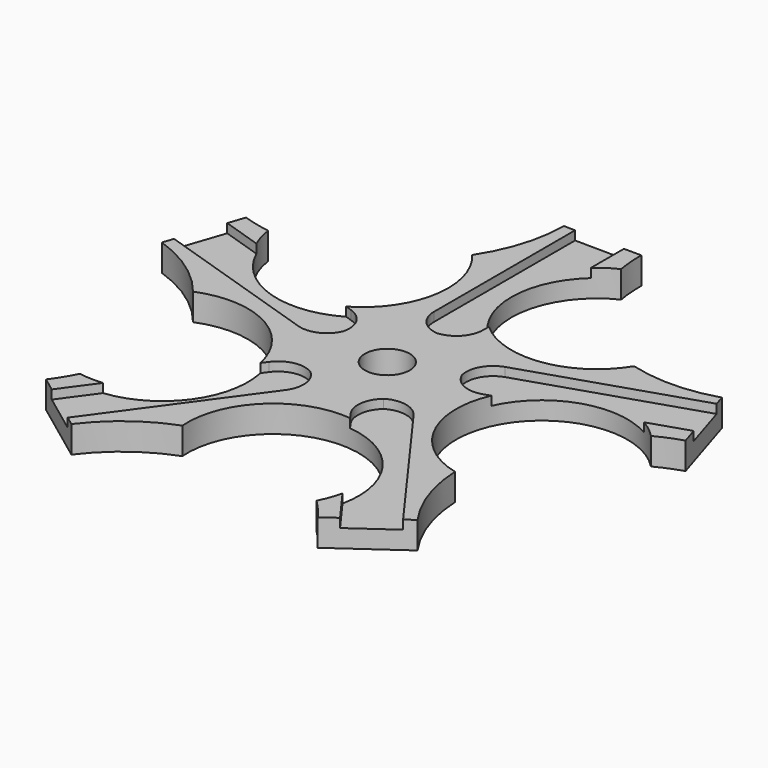
from build123d import *

# Parameters (mm, degrees)
F0_R        = 2.5
F1_DEPTH    = 3
F3_DEPTH    = 1
F4_T1_DEPTH = 1


# Not quite as in the source:
# - a fillet or chamfer that OpenCascade refuses, or shapes differently, is made with other operations: its cross-section is extruded or revolved along the edge and cut away or added


with BuildPart() as f1:
    # F0 (on Top) → F1 (new body)
    with BuildSketch(Plane.XY):
        with BuildLine():
            Line((42.1995138221, 67.0275468757), (33.4926469464, 67.1294207869))
            ThreePointArc((33.4926469464, 67.1294207869), (32.7404851321, 62.3046461892), (30.658157874, 57.8878475177))
            ThreePointArc((30.658157874, 57.8878475177), (27.294204133, 42.9798709067), (13.9152540739, 50.3668626301))
            ThreePointArc((13.9152540739, 50.3668626301), (12.375918121, 50.6607466073), (10.86986377, 51.0940170307))
            Line((10.86986377, 51.0940170307), (8.0824060906, 42.844775322))
            ThreePointArc((8.0824060906, 42.844775322), (12.4386086282, 40.6384895823), (15.9957592753, 37.2932128243))
            ThreePointArc((15.9957592753, 37.2932128243), (29.1345687017, 29.4870845738), (17.9747991522, 19.0456529188))
            ThreePointArc((17.9747991522, 19.0456529188), (17.2196179112, 17.6724725733), (16.3421568627, 16.3740176929))
            Line((16.3421568627, 16.3740176929), (23.3262801503, 11.1738320243))
            ThreePointArc((23.3262801503, 11.1738320243), (26.7707231948, 14.6350470461), (31.0514904559, 16.9843509793))
            ThreePointArc((31.0514904559, 16.9843509793), (42.5356749941, 27.0678750109), (49.017508165, 13.2277236335))
            ThreePointArc((49.017508165, 13.2277236335), (50.0901164433, 12.0851675302), (51.0538700425, 10.8494078578))
            Line((51.0538700425, 10.8494078578), (58.1577532953, 15.8847580755))
            ThreePointArc((58.1577532953, 15.8847580755), (55.9303336315, 20.230192341), (55.0188426496, 25.0274187796))
            ThreePointArc((55.0188426496, 25.0274187796), (48.977649601, 39.065507608), (64.1434123595, 40.9532553024))
            ThreePointArc((64.1434123595, 40.9532553024), (65.5615019731, 41.620297142), (67.0345955027, 42.1550105429))
            Line((67.0345955027, 42.1550105429), (64.4409135174, 50.4672137913))
            ThreePointArc((64.4409135174, 50.4672137913), (59.6198494134, 49.6916248415), (54.7757497452, 50.307169899))
            ThreePointArc((54.7757497452, 50.307169899), (39.5579025703, 48.8996619005), (42.4490262494, 63.9065055152))
            ThreePointArc((42.4490262494, 63.9065055152), (42.2528455514, 65.4613161473), (42.1995138221, 67.0275468757))
        make_face()
        with Locations((37.5, 37.5)):
            Circle(F0_R, mode=Mode.SUBTRACT)
    extrude(amount=F1_DEPTH)

    # F2 (on face) → F3 (cut)
    with BuildSketch(Plane.XY.offset(3)):
        Polygon((40.25, 67.1147092408), (34.75, 67.1147092408), (40.25, 67.0503569865), align=None)
        with BuildLine():
            Line((31.7569283434, 42.2575582148), (28.1635644564, 43.4251129174))
            ThreePointArc((28.1635644564, 43.4251129174), (20.4254111601, 42.6084822131), (14.6451171229, 47.8175227185))
            Line((14.6451171229, 47.8175227185), (10.2457371637, 49.2469679185))
            Line((10.2457371637, 49.2469679185), (8.4849410638, 44.0360430191))
            Line((8.4849410638, 44.0360430191), (30.0573348743, 37.0267473751))
            Line((30.0573348743, 37.0267473751), (31.7569283434, 42.2575582148))
        make_face()
        with BuildLine():
            Line((31.2005865164, 33.5081806175), (28.9797655003, 30.4514827223))
            ThreePointArc((28.9797655003, 30.4514827223), (27.3652065793, 22.8397088401), (20.6249055731, 18.9520045705))
            Line((20.6249055731, 18.9520045705), (17.9059392288, 15.2096684519))
            Line((17.9059392288, 15.2096684519), (22.3177073919, 11.9247874969))
            Line((22.3177073919, 11.9247874969), (35.6501799855, 30.2753617299))
            Line((35.6501799855, 30.2753617299), (31.2005865164, 33.5081806175))
        make_face()
        with BuildLine():
            Line((52.6444673021, 11.9768495643), (57.1318860772, 15.1576063845))
            Line((57.1318860772, 15.1576063845), (43.7994134836, 33.5081806175))
            Line((43.7994134836, 33.5081806175), (39.3498200145, 30.2753617299))
            Line((39.3498200145, 30.2753617299), (41.5706410307, 27.2186638347))
            ThreePointArc((41.5706410307, 27.2186638347), (48.3109420369, 23.3309595651), (49.9255009579, 15.7191856828))
            Line((49.9255009579, 15.7191856828), (52.6444673021, 11.9768495643))
        make_face()
        with BuildLine():
            Line((66.4538563054, 44.0161570789), (64.8154654671, 49.2668538587))
            Line((64.8154654671, 49.2668538587), (43.2430716566, 42.2575582148))
            Line((43.2430716566, 42.2575582148), (44.9426651257, 37.0267473751))
            Line((44.9426651257, 37.0267473751), (48.5360290127, 38.1943020778))
            ThreePointArc((48.5360290127, 38.1943020778), (54.3163230499, 43.4033425831), (62.0544763461, 42.5867118789))
            Line((62.0544763461, 42.5867118789), (66.4538563054, 44.0161570789))
        make_face()
        with BuildLine():
            Line((34.75, 44.4321520627), (37.5, 44.4321520627))
            Line((37.5, 44.4321520627), (40.25, 44.4321520627))
            Line((40.25, 44.4321520627), (40.25, 48.2104384478))
            ThreePointArc((40.25, 48.2104384478), (37.0821171737, 55.3175067985), (40.25, 62.4245751493))
            Line((40.25, 62.4245751493), (40.25, 67.0503569865))
            Line((40.25, 67.0503569865), (34.75, 67.1147092408))
            Line((34.75, 67.1147092408), (34.75, 44.4321520627))
        make_face()
    extrude(amount=-F3_DEPTH, mode=Mode.SUBTRACT)

    # F4: fillet of radius 3 on 10 edges, made by hand

    # F4_s2 → F4_t1 (join)
    with BuildSketch(Plane.XY.offset(2)):
        with BuildLine():
            ThreePointArc((37.25, 44.4321520627), (39.3713203436, 45.3108317191), (40.25, 47.4321520627))
            Line((40.25, 47.4321520627), (40.25, 44.4321520627))
            Line((40.25, 44.4321520627), (37.25, 44.4321520627))
        make_face()
        with BuildLine():
            ThreePointArc((34.75, 47.4321520627), (35.6286796564, 45.3108317191), (37.75, 44.4321520627))
            Line((37.75, 44.4321520627), (34.75, 44.4321520627))
            Line((34.75, 44.4321520627), (34.75, 47.4321520627))
        make_face()
        with BuildLine():
            ThreePointArc((30.8298773603, 39.4043886659), (30.6497273839, 41.6934111482), (28.9037587945, 43.1846091979))
            Line((28.9037587945, 43.1846091979), (31.7569283434, 42.2575582148))
            Line((31.7569283434, 42.2575582148), (30.8298773603, 39.4043886659))
        make_face()
        with BuildLine():
            ThreePointArc((27.2041653254, 37.9537983583), (29.4931878078, 38.1339483346), (30.9843858575, 39.879916924))
            Line((30.9843858575, 39.879916924), (30.0573348743, 37.0267473751))
            Line((30.0573348743, 37.0267473751), (27.2041653254, 37.9537983583))
        make_face()
        with BuildLine():
            ThreePointArc((33.6276374995, 31.7448248606), (31.3949783475, 32.2808388993), (29.4372307595, 31.0811296344))
            Line((29.4372307595, 31.0811296344), (31.2005865164, 33.5081806175))
            Line((31.2005865164, 33.5081806175), (33.6276374995, 31.7448248606))
        make_face()
        with BuildLine():
            ThreePointArc((33.8868242286, 27.8483107468), (34.4228382672, 30.0809698988), (33.2231290023, 32.0387174868))
            Line((33.2231290023, 32.0387174868), (35.6501799855, 30.2753617299))
            Line((35.6501799855, 30.2753617299), (33.8868242286, 27.8483107468))
        make_face()
        with BuildLine():
            ThreePointArc((41.1131757714, 27.8483107468), (40.5771617328, 30.0809698988), (41.7768709977, 32.0387174868))
            Line((41.7768709977, 32.0387174868), (39.3498200145, 30.2753617299))
            Line((39.3498200145, 30.2753617299), (41.1131757714, 27.8483107468))
        make_face()
        with BuildLine():
            ThreePointArc((45.5627692405, 31.0811296344), (43.6050216525, 32.2808388993), (41.3723625005, 31.7448248606))
            Line((41.3723625005, 31.7448248606), (43.7994134836, 33.5081806175))
            Line((43.7994134836, 33.5081806175), (45.5627692405, 31.0811296344))
        make_face()
        with BuildLine():
            ThreePointArc((44.0156141425, 39.879916924), (45.5068121922, 38.1339483346), (47.7958346746, 37.9537983583))
            Line((47.7958346746, 37.9537983583), (44.9426651257, 37.0267473751))
            Line((44.9426651257, 37.0267473751), (44.0156141425, 39.879916924))
        make_face()
        with BuildLine():
            ThreePointArc((46.0962412055, 43.1846091979), (44.3502726161, 41.6934111482), (44.1701226397, 39.4043886659))
            Line((44.1701226397, 39.4043886659), (43.2430716566, 42.2575582148))
            Line((43.2430716566, 42.2575582148), (46.0962412055, 43.1846091979))
        make_face()
    extrude(amount=F4_T1_DEPTH)


solid = f1.part
